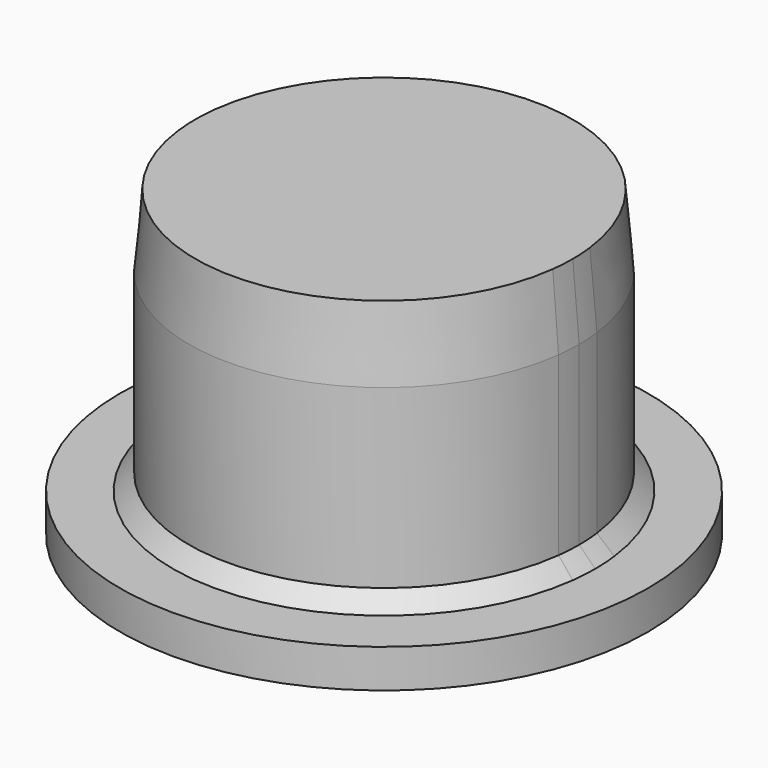
from build123d import *

# Parameters (mm, degrees)
F1_DEPTH = 9.5
F2_T     = -0.8
F0_R     = 8.25
F3_DEPTH = 1.2
F4_SIZE2 = 2.2860104606
F4_SIZE  = 0.2
F5_SIZE  = 0.5


with BuildPart() as f1:
    # F0 (on Top) → F1 (new body)
    with BuildSketch(Plane.XY):
        with BuildLine():
            ThreePointArc((6.0537178659, -0.75), (6.0884184721, -0.3757133335), (6.1, 0))
            ThreePointArc((6.1, 0), (6.0884184721, 0.3757133335), (6.0537178659, 0.75))
            Line((6.0537178659, 0.75), (-6.0537178659, 0.75))
            ThreePointArc((-6.0537178659, 0.75), (-6.1, 0), (-6.0537178659, -0.75))
            Line((-6.0537178659, -0.75), (6.0537178659, -0.75))
        make_face()
        with BuildLine():
            Line((-6.0537178659, 0.75), (6.0537178659, 0.75))
            ThreePointArc((6.0537178659, 0.75), (0, 6.1), (-6.0537178659, 0.75))
        make_face()
        with BuildLine():
            ThreePointArc((-6.0537178659, -0.75), (0, -6.1), (6.0537178659, -0.75))
            Line((6.0537178659, -0.75), (-6.0537178659, -0.75))
        make_face()
    extrude(amount=F1_DEPTH)

    # F2
    f2_openings = [f1.faces().sort_by_distance(p)[0] for p in [
        (0, 0, 0),
    ]]
    offset(amount=F2_T, openings=f2_openings)

    # F0 (on Top) → F3 (join)
    with BuildSketch(Plane.XY):
        Circle(F0_R)
        with BuildLine():
            ThreePointArc((-6.0537178659, 0.75), (0, 6.1), (6.0537178659, 0.75))
            Line((6.0537178659, 0.75), (7.5, 0.75))
            Line((7.5, 0.75), (7.5, -0.75))
            Line((7.5, -0.75), (6.0537178659, -0.75))
            ThreePointArc((6.0537178659, -0.75), (0, -6.1), (-6.0537178659, -0.75))
            Line((-6.0537178659, -0.75), (-7.5, -0.75))
            Line((-7.5, -0.75), (-7.5, 0.75))
            Line((-7.5, 0.75), (-6.0537178659, 0.75))
        make_face(mode=Mode.SUBTRACT)
        with BuildLine():
            ThreePointArc((6.0537178659, -0.75), (6.0884184721, -0.3757133335), (6.1, 0))
            ThreePointArc((6.1, 0), (6.0884184721, 0.3757133335), (6.0537178659, 0.75))
            Line((6.0537178659, 0.75), (-6.0537178659, 0.75))
            ThreePointArc((-6.0537178659, 0.75), (-6.1, 0), (-6.0537178659, -0.75))
            Line((-6.0537178659, -0.75), (6.0537178659, -0.75))
        make_face()
        with BuildLine():
            ThreePointArc((6.0537178659, 0.75), (6.0884184721, 0.3757133335), (6.1, 0))
            ThreePointArc((6.1, 0), (6.0884184721, -0.3757133335), (6.0537178659, -0.75))
            Line((6.0537178659, -0.75), (7.5, -0.75))
            Line((7.5, -0.75), (7.5, 0.75))
            Line((7.5, 0.75), (6.0537178659, 0.75))
        make_face()
        with BuildLine():
            ThreePointArc((-6.0537178659, -0.75), (-6.1, 0), (-6.0537178659, 0.75))
            Line((-6.0537178659, 0.75), (-7.5, 0.75))
            Line((-7.5, 0.75), (-7.5, -0.75))
            Line((-7.5, -0.75), (-6.0537178659, -0.75))
        make_face()
    extrude(amount=F3_DEPTH)

    # F4
    f4_edges = [f1.edges().sort_by_distance(p)[0] for p in [
        (6.053718, 0.75, 9.5),
    ]]
    f4_side = f1.faces().sort_by_distance((0, 0, 9.5))[0]
    chamfer(f4_edges, length=F4_SIZE, length2=F4_SIZE2, reference=f4_side)

    # F5
    f5_edges = [f1.edges().sort_by_distance(p)[0] for p in [
        (6.053718, 0.75, 1.2),
    ]]
    chamfer(f5_edges, length=F5_SIZE)


solid = f1.part
